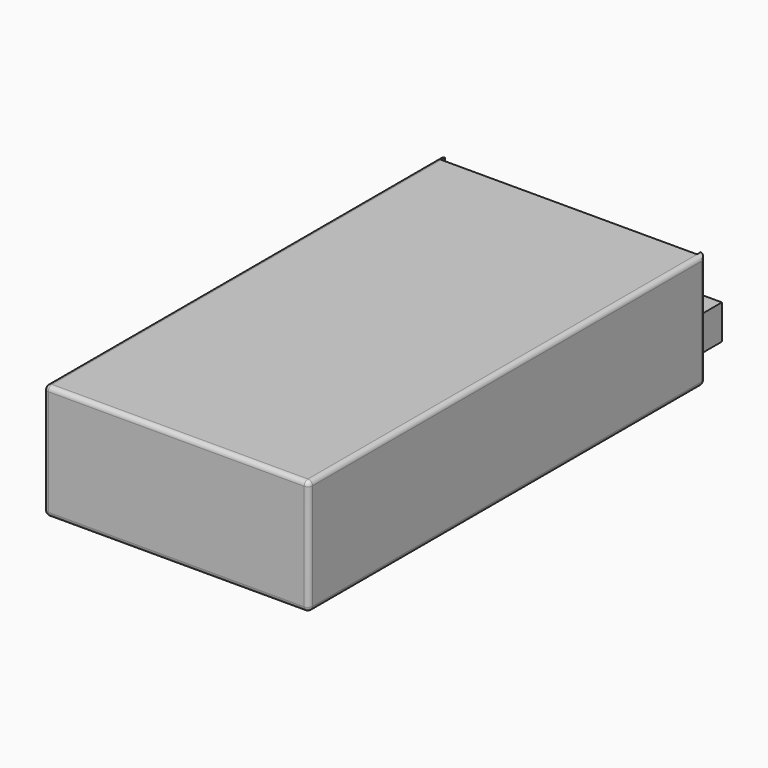
from build123d import *

# Parameters (mm, degrees)
F0_W     = 115
F0_H     = 215
F1_DEPTH = 25
F2_W     = 111
F2_H     = 41.5
F3_DEPTH = 2
F4_W     = 88.5
F4_H     = 15
F5_DEPTH = 16
F6_R     = 1.99999


# Not quite as in the source:
# - a fillet or chamfer is up to 0.001 mm smaller than in the source, because OpenCascade refuses the exact size


with BuildPart() as f1:
    # F0 (on Top) → F1 (new body, symmetric)
    with BuildSketch(Plane.XY):
        Rectangle(F0_W, F0_H)
    extrude(amount=F1_DEPTH, both=True)

    # F2 (on face) → F3 (cut)
    with BuildSketch(Plane(origin=(0, 107.5, 0), x_dir=(-1, 0, 0), z_dir=(0, 1, 0))):
        with Locations((0, 4.25)):
            Rectangle(F2_W, F2_H)
    extrude(amount=-F3_DEPTH, mode=Mode.SUBTRACT)

    # F4 (on face) → F5 (join)
    with BuildSketch(Plane(origin=(0, 105.5, 0), x_dir=(-1, 0, 0), z_dir=(0, 1, 0))):
        with Locations((-9.25, -8)):
            Rectangle(F4_W, F4_H)
    extrude(amount=F5_DEPTH)

    # F6 (radius 2 in the source; OpenCascade refuses exactly that, so slightly less here)
    f6_edges = [f1.edges().sort_by_distance(p)[0] for p in [
        (-57.5, 107.5, 0),
        (-57.5, 0, -25),
        (-57.5, -107.5, 0),
        (-57.5, 0, 25),
        (57.5, 0, -25),
        (57.5, 107.5, 0),
        (57.5, 0, 25),
        (57.5, -107.5, 0),
        (0, 107.5, -25),
        (0, -107.5, -25),
        (0, -107.5, 25),
    ]]
    fillet(f6_edges, radius=F6_R)


solid = f1.part
